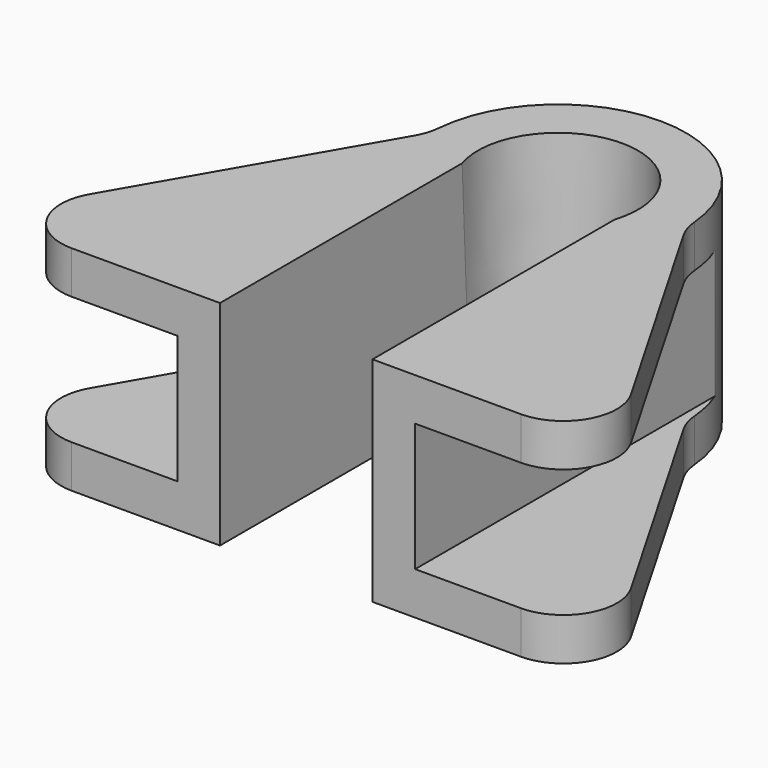
from build123d import *

# Parameters (mm, degrees)
F3_R      = 24
F4_DEPTH  = 40
F0_R      = 15
F2_R      = 14.5
F7_DEPTH  = 40.0010001
F9_DEPTH  = 40
F10_W     = 37.1058717763
F10_H     = 24
F11_DEPTH = 85.2906296813
F12_R     = 10
F13_R     = 10


# Not quite as in the source:
# - a pattern or mirror of a feature is missing from the dataset's text; its kind, count and spacing are read off the source's solid


with BuildPart() as f4:
    # F3 (on Top) → F4 (new body)
    with BuildSketch(Plane.XY):
        Circle(F3_R)
    extrude(amount=-F4_DEPTH)

    # F0 (on Top) → F5 section 0
    with BuildSketch(Plane.XY):
        Circle(F0_R)
    # F2 (on offset) → F5 section 1
    with BuildSketch(Plane.XY.offset(-40)):
        Circle(F2_R)
    loft(mode=Mode.SUBTRACT)

    # F6 (on face) → F7 (cut, through all)
    with BuildSketch(Plane.XY):
        with BuildLine():
            Line((-14.2797124187, -4.5923646676), (-14.2797124187, -19.2896296813))
            ThreePointArc((-14.2797124187, -19.2896296813), (0, -24), (14.2797124187, -19.2896296813))
            Line((14.2797124187, -19.2896296813), (14.2797124187, -4.5923646676))
            ThreePointArc((14.2797124187, -4.5923646676), (0, -15), (-14.2797124187, -4.5923646676))
        make_face()
        with BuildLine():
            Line((-14.2797124187, -2.5178985762), (-14.2797124187, -4.5923646676))
            ThreePointArc((-14.2797124187, -4.5923646676), (0, -15), (14.2797124187, -4.5923646676))
            Line((14.2797124187, -4.5923646676), (14.2797124187, -2.5178985762))
            ThreePointArc((14.2797124187, -2.5178985762), (0, -14.5), (-14.2797124187, -2.5178985762))
        make_face()
    extrude(amount=-F7_DEPTH, mode=Mode.SUBTRACT)

    # F8 (on face) → F9 (join)
    with BuildSketch(Plane.XY):
        with BuildLine():
            Line((-14.2797124187, -61.2896296813), (-14.2797124187, -19.2896296813))
            ThreePointArc((-14.2797124187, -19.2896296813), (-21.4326048119, -10.8001597662), (-24, 0))
            Line((-24, 0), (-59.385584195, -61.2896296813))
            Line((-59.385584195, -61.2896296813), (-14.2797124187, -61.2896296813))
        make_face()
        with BuildLine():
            ThreePointArc((24, 0), (21.4326048119, -10.8001597662), (14.2797124187, -19.2896296813))
            Line((14.2797124187, -19.2896296813), (14.2797124187, -61.2896296813))
            Line((14.2797124187, -61.2896296813), (59.385584195, -61.2896296813))
            Line((59.385584195, -61.2896296813), (24, 0))
        make_face()
    extrude(amount=-F9_DEPTH)

    # F10 (on face) → F11 (cut, through all)
    with BuildSketch(Plane.XZ.offset(61.2896296813)):
        with Locations((-40.8326483068, -20)):
            Rectangle(F10_W, F10_H)
    f11 = extrude(amount=-F11_DEPTH, mode=Mode.SUBTRACT)

    # F11_copies: F11 across plane
    add(f11.mirror(Plane(origin=(0, 0, 0), x_dir=(0, 0, 1), z_dir=(1, 0, 0))), mode=Mode.SUBTRACT)

    # F12
    f12_edges = [f4.edges().sort_by_distance(p)[0] for p in [
        (-59.385584, -61.28963, -4),
        (-59.385584, -61.28963, -36),
        (-24, 0, -4),
        (-24, 0, -36),
    ]]
    fillet(f12_edges, radius=F12_R)

    # F13
    f13_edges = [f4.edges().sort_by_distance(p)[0] for p in [
        (59.385584, -61.28963, -4),
        (59.385584, -61.28963, -36),
        (24, 0, -4),
        (24, 0, -36),
    ]]
    fillet(f13_edges, radius=F13_R)


solid = f4.part
